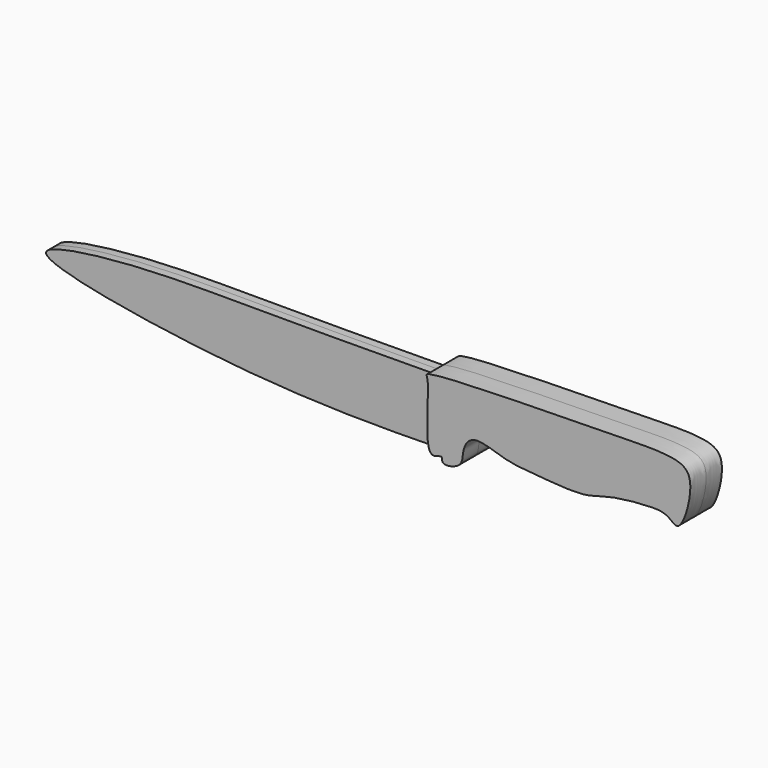
from build123d import *

# Parameters (mm, degrees)
F1_DEPTH = 3.175
F2_DEPTH = 1.27


# Not quite as in the source:
# - a feature names something its author has since deleted; it is built from what else it names


with BuildPart() as f1:
    # F0 (on Front) → F1 (new body, symmetric)
    with BuildSketch(Plane.XZ):
        with BuildLine():
            add(Edge.make_bspline(
                [(11.1371772364, -5.7724104263), (9.8633713226, -4.8247675972), (10.8286121975, 2.430426847), (10.5211958289, 4.4528897852)],
                knots=[0, 0, 0, 0, 0.0815389543, 0.0815389543, 0.0815389543, 0.0815389543], degree=3))
            add(Edge.make_bspline(
                [(10.5211958289, 4.4528897852), (10.4320001713, 5.0396995004), (9.095258314, 6.035740183), (40.8754630173, 6.3489667059), (49.4732836858, 6.7059004077), (53.9141732937, 4.8849321277), (51.2551424038, -4.6497415166), (49.1602833702, -1.8049068404), (45.6544543574, -1.7344569531), (39.5328517037, -2.3574791172), (35.6695305458, -3.9894974099), (28.3375317285, -3.2304414165), (23.1238506636, -3.006341842), (17.7764330461, -0.6323517487), (15.9945351129, -3.5138109738), (16.3558266304, -6.2240997641), (12.5395223866, -6.9615509617), (13.0929226507, -5.1063664031), (11.6415866883, -6.1476638263), (11.1371772364, -5.7724104263)],
                knots=[0.0815389543, 0.0815389543, 0.0815389543, 0.0815389543, 0.1051971631, 0.2426160928, 0.3252988962, 0.3715422501, 0.4407534093, 0.4745888175, 0.5221447944, 0.5849718523, 0.6378191575, 0.7053502486, 0.7662538979, 0.8233650841, 0.8639654446, 0.9038799254, 0.9452238609, 0.9677117065, 1, 1, 1, 1], degree=3))
        make_face()
    extrude(amount=F1_DEPTH, both=True)


with BuildPart() as f2:
    # F0 (on Front) → F2 (new body, symmetric)
    with BuildSketch(Plane.XZ):
        with BuildLine():
            add(Edge.make_bspline(
                [(10.5211958289, 4.4528897852), (0.6484246724, 4.3666230029), (-18.1448455868, 4.2309187987), (-39.1976188833, 4.5061369229), (-59.7700102657, 1.1575986861), (-29.4145074355, -4.5774135742), (-5.2471983118, -6.0617033098), (6.2329714332, -5.8526263684), (11.1371772364, -5.7724104263)],
                knots=[0, 0, 0, 0, 0.1968998186, 0.3748002279, 0.4950748533, 0.6612203133, 0.8552686491, 1, 1, 1, 1], degree=3))
            add(Edge.make_bspline(
                [(11.1371772364, -5.7724104263), (9.8633713226, -4.8247675972), (10.8286121975, 2.430426847), (10.5211958289, 4.4528897852)],
                knots=[0, 0, 0, 0, 0.0815389543, 0.0815389543, 0.0815389543, 0.0815389543], degree=3))
        make_face()
    extrude(amount=F2_DEPTH, both=True)


solid = Compound([f1.part, f2.part])
